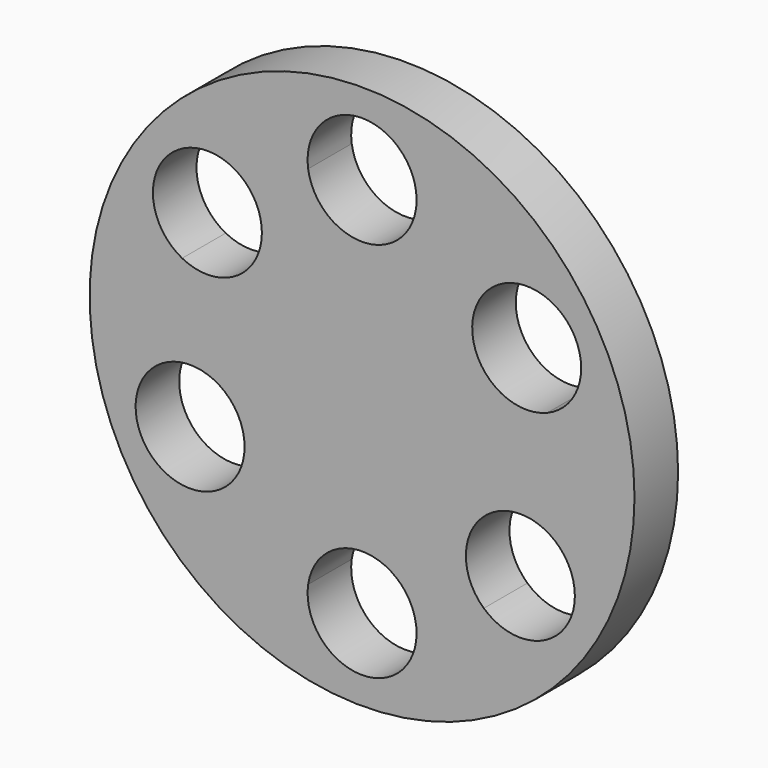
from build123d import *

# Parameters (mm, degrees)
F0_R     = 10
F1_DEPTH = 2
F3_DEPTH = 2.001


with BuildPart() as f1:
    # F0 (on Front) → F1 (new body)
    with BuildSketch(Plane.XZ):
        Circle(F0_R)
    extrude(amount=F1_DEPTH)

    # F2 (on face) → F3 (cut, through all)
    with BuildSketch(Plane.XZ.offset(2)):
        with BuildLine():
            ThreePointArc((4.795326069, 5.0994948663), (4.3154664556, 2.525222618), (6.7947838404, 1.6825315934))
            ThreePointArc((6.7947838404, 1.6825315934), (6.0416530379, 3.5353116652), (4.795326069, 5.0994948663))
        make_face()
        with BuildLine():
            ThreePointArc((4.795326069, 5.0994948663), (6.0416530379, 3.5353116652), (6.7947838404, 1.6825315934))
            ThreePointArc((6.7947838404, 1.6825315934), (7.700909137, 2.4186786917), (8.0416530379, 3.5353116652))
            ThreePointArc((8.0416530379, 3.5353116652), (6.9097964771, 5.3370682994), (4.795326069, 5.0994948663))
        make_face()
        with BuildLine():
            ThreePointArc((7.8100628501, -3.9042502068), (7.5032590313, -2.8397847578), (6.6769761581, -2.1019013736))
            ThreePointArc((6.6769761581, -2.1019013736), (5.8100628501, -3.9042502068), (4.4688586973, -5.3878847374))
            ThreePointArc((4.4688586973, -5.3878847374), (6.6217252474, -5.7321463069), (7.8100628501, -3.9042502068))
        make_face()
        with BuildLine():
            ThreePointArc((4.4688586973, -5.3878847374), (5.8100628501, -3.9042502068), (6.6769761581, -2.1019013736))
            ThreePointArc((6.6769761581, -2.1019013736), (4.150044893, -2.7887501477), (4.4688586973, -5.3878847374))
        make_face()
        with BuildLine():
            ThreePointArc((-1.9794866372, 6.7142857143), (0, 5), (1.9794866372, 6.7142857143))
            ThreePointArc((1.9794866372, 6.7142857143), (0, 7), (-1.9794866372, 6.7142857143))
        make_face()
        with BuildLine():
            ThreePointArc((-1.9794866372, 6.7142857143), (0, 7), (1.9794866372, 6.7142857143))
            ThreePointArc((1.9794866372, 6.7142857143), (1.9948650674, 6.8567751321), (2, 7))
            ThreePointArc((2, 7), (-0.1432248679, 8.9948650674), (-1.9794866372, 6.7142857143))
        make_face()
        with BuildLine():
            ThreePointArc((2, -7), (1.9948650674, -6.8567751321), (1.9794866372, -6.7142857143))
            ThreePointArc((1.9794866372, -6.7142857143), (0, -7), (-1.9794866372, -6.7142857143))
            ThreePointArc((-1.9794866372, -6.7142857143), (-0.1432248679, -8.9948650674), (2, -7))
        make_face()
        with BuildLine():
            ThreePointArc((-1.9794866372, -6.7142857143), (0, -7), (1.9794866372, -6.7142857143))
            ThreePointArc((1.9794866372, -6.7142857143), (0, -5), (-1.9794866372, -6.7142857143))
        make_face()
        with BuildLine():
            ThreePointArc((-3.6779306672, 4.0940326499), (-3.8368770547, 4.8753914638), (-4.2884522632, 5.5325561168))
            ThreePointArc((-4.2884522632, 5.5325561168), (-5.6779306672, 4.0940326499), (-6.6039045269, 2.321302436))
            ThreePointArc((-6.6039045269, 2.321302436), (-4.6415783428, 2.3834848255), (-3.6779306672, 4.0940326499))
        make_face()
        with BuildLine():
            ThreePointArc((-6.6039045269, 2.321302436), (-5.6779306672, 4.0940326499), (-4.2884522632, 5.5325561168))
            ThreePointArc((-4.2884522632, 5.5325561168), (-7.3001965721, 5.2637562642), (-6.6039045269, 2.321302436))
        make_face()
        with BuildLine():
            ThreePointArc((-6.9101605699, -1.1178912729), (-8.1154178378, -3.891014433), (-5.1985581087, -4.6877493096))
            ThreePointArc((-5.1985581087, -4.6877493096), (-6.3119916516, -3.026344559), (-6.9101605699, -1.1178912729))
        make_face()
        with BuildLine():
            ThreePointArc((-6.9101605699, -1.1178912729), (-6.3119916516, -3.026344559), (-5.1985581087, -4.6877493096))
            ThreePointArc((-5.1985581087, -4.6877493096), (-4.5474992195, -3.9679211396), (-4.3119916516, -3.026344559))
            ThreePointArc((-4.3119916516, -3.026344559), (-5.1280021746, -1.4144609037), (-6.9101605699, -1.1178912729))
        make_face()
    extrude(amount=-F3_DEPTH, mode=Mode.SUBTRACT)


solid = f1.part
